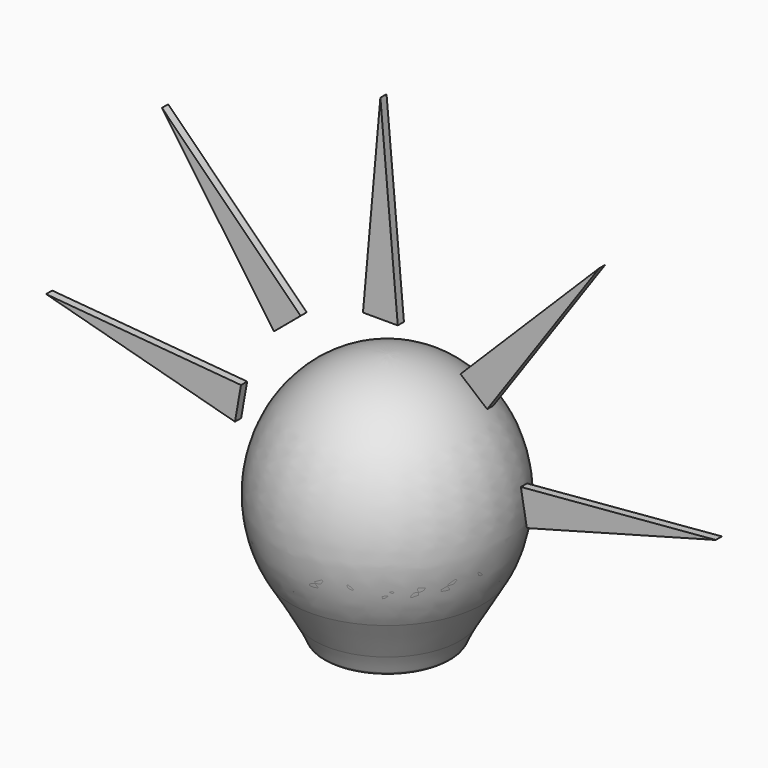
from build123d import *

# Parameters (mm, degrees)
F2_T     = 0.1
F4_DEPTH = 2
F6_COUNT = 3
F6_ANGLE = 80
F7_COUNT = 3
F7_ANGLE = 80


# Not quite as in the source:
# - a shell that OpenCascade refuses in one call is made with other operations: the cavity is built on its own and cut out


with BuildPart() as f1:
    # F0 (on Front) → F1 (revolve)
    with BuildSketch(Plane.XZ):
        with BuildLine():
            Line((-15.4683816494, 0), (0, 0))
            Line((0, 0), (0, 65))
            add(Edge.make_bspline(
                [(0, 65), (-53.6115006556, 65), (-24.9198123266, 15.8303619511)],
                knots=[0, 0, 0, 2.135514613, 2.135514613, 2.135514613], degree=2, weights=[1, 0.4820903118, 1]))
            Line((-24.9198123266, 15.8303619511), (-18.8718817936, 5.4658775806))
            ThreePointArc((-18.8718817936, 5.4658775806), (-17.6054522133, 3.1172637552), (-16.5, 0.6887238263))
            ThreePointArc((-16.5, 0.6887238263), (-16.0885785799, 0.188002688), (-15.4683816494, 0))
        make_face()
    revolve(axis=Axis((0, 0, 32.5), (0, 0, 1)))

    # F2: shell of thickness 0.1, made by hand


with BuildPart() as f2_core1:
    # F2_t2: copy of F1
    add(f1.part)

    # the walls: a layer under each face that stays
    f2_faces = [f2_core1.faces().sort_by_distance(p)[0] for p in [
        (17.6054522133, 0, 3.1172637552),
        (16.0885785799, 0, 0.188002688),
        (25.8455850667, 0, 48.4120641443),
        (21.8958470601, 0, 10.6481197659),
    ]]
    thicken(f2_faces, amount=-F2_T, mode=Mode.SUBTRACT)


with BuildPart() as f1_1:
    add(f1.part)

    # what is left inside the walls is the cavity
    f2_cavity = [f2_core1.part.solids().sort_by_distance(p)[0] for p in [
        (18.451865, 0, 57.827147),
    ]]
    add(f2_cavity, mode=Mode.SUBTRACT)


with BuildPart() as f4:
    # F3 (on Front) → F4 (new body)
    with BuildSketch(Plane.XZ):
        Polygon((4.3439801882, 73.6905180782), (-0.1720996806, 124.2893819253), (-4.6881795495, 73.6905180782), align=None)
    extrude(amount=F4_DEPTH)


with BuildPart() as f6_1:
    # F6: instance of F4
    add(f4.part.rotate(Axis((0, 0, 36), (0, 1, 0)), 1 * F6_ANGLE / (F6_COUNT - 1)))


with BuildPart() as f6_2:
    # F6: instance of F4
    add(f4.part.rotate(Axis((0, 0, 36), (0, 1, 0)), 2 * F6_ANGLE / (F6_COUNT - 1)))


with BuildPart() as f7_1:
    # F7: instance of F4
    add(f4.part.rotate(Axis((0, 0, 36), (0, -1, 0)), 1 * F7_ANGLE / (F7_COUNT - 1)))


with BuildPart() as f7_2:
    # F7: instance of F4
    add(f4.part.rotate(Axis((0, 0, 36), (0, -1, 0)), 2 * F7_ANGLE / (F7_COUNT - 1)))


solid = Compound([f1_1.part, f4.part, f6_1.part, f6_2.part, f7_1.part, f7_2.part])
